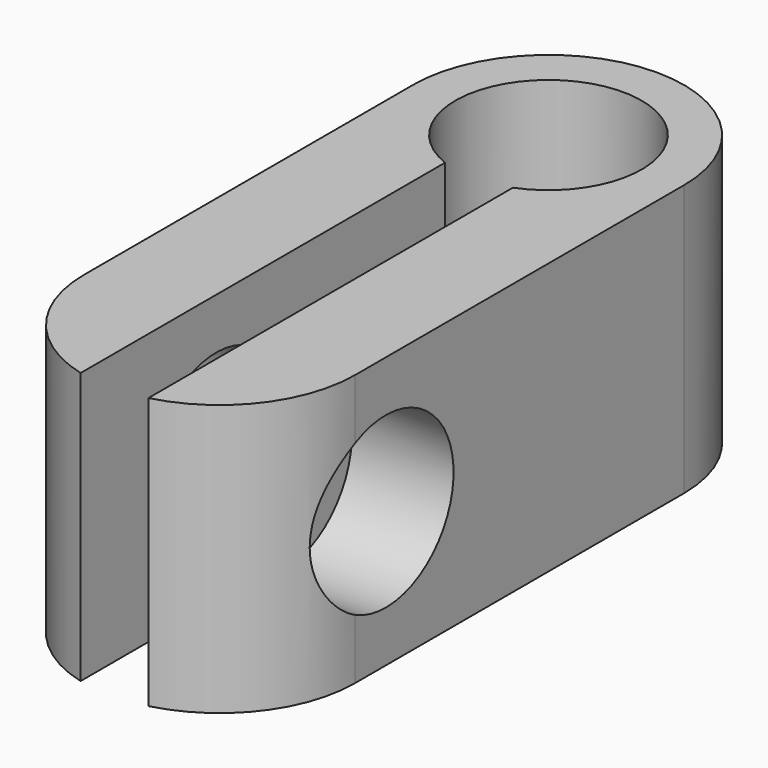
from build123d import *

# Parameters (mm, degrees)
F0_W        = 8
F0_H        = 8
F1_DEPTH    = 20
F2_R        = 3.99999
F4_DEPTH    = 25
F6_T1_DEPTH = 27.364916731
F5_R        = 2.5
F7_DEPTH    = 25


# Not quite as in the source:
# - a fillet or chamfer that OpenCascade refuses, or shapes differently, is made with other operations: its cross-section is extruded or revolved along the edge and cut away or added
# - a fillet or chamfer is up to 0.001 mm smaller than in the source, because OpenCascade refuses the exact size


with BuildPart() as f1:
    # F0 (on Front) → F1 (new body)
    with BuildSketch(Plane.XZ):
        with Locations((4, 4)):
            Rectangle(F0_W, F0_H)
    extrude(amount=F1_DEPTH)

    # F2 (radius 4 in the source; OpenCascade refuses exactly that, so slightly less here)
    f2_edges = [f1.edges().sort_by_distance(p)[0] for p in [
        (8, 0, 4),
        (0, 0, 4),
    ]]
    fillet(f2_edges, radius=F2_R)

    # F3 (on face) → F4 (cut)
    with BuildSketch(Plane.XY.offset(8)):
        with BuildLine():
            Line((5, -20), (5, -6.5617376915))
            ThreePointArc((5, -6.5617376915), (4, -1.25), (3, -6.5617376915))
            Line((3, -6.5617376915), (3, -20))
            Line((3, -20), (4, -20))
            Line((4, -20), (5, -20))
        make_face()
    extrude(amount=-F4_DEPTH, mode=Mode.SUBTRACT)

    # F6: fillet of radius 4 on 2 edges, made by hand

    # F6_s2 → F6_t1 (cut)
    with BuildSketch(Plane.XY.offset(-9.6824583655)):
        with BuildLine():
            ThreePointArc((0, -16.1270166538), (0.8377223398, -18.5765063966), (3, -20))
            Line((3, -20), (0, -20))
            Line((0, -20), (0, -16.1270166538))
        make_face()
        with BuildLine():
            ThreePointArc((5, -20), (7.1622776602, -18.5765063966), (8, -16.1270166538))
            Line((8, -16.1270166538), (8, -20))
            Line((8, -20), (5, -20))
        make_face()
    extrude(amount=F6_T1_DEPTH, mode=Mode.SUBTRACT)

    # F5 (on face) → F7 (cut)
    with BuildSketch(Plane(origin=(0, 0, 0), x_dir=(0, -1, 0), z_dir=(-1, 0, 0))):
        with Locations((15, 4)):
            Circle(F5_R)
    extrude(amount=-F7_DEPTH, mode=Mode.SUBTRACT)


solid = f1.part
